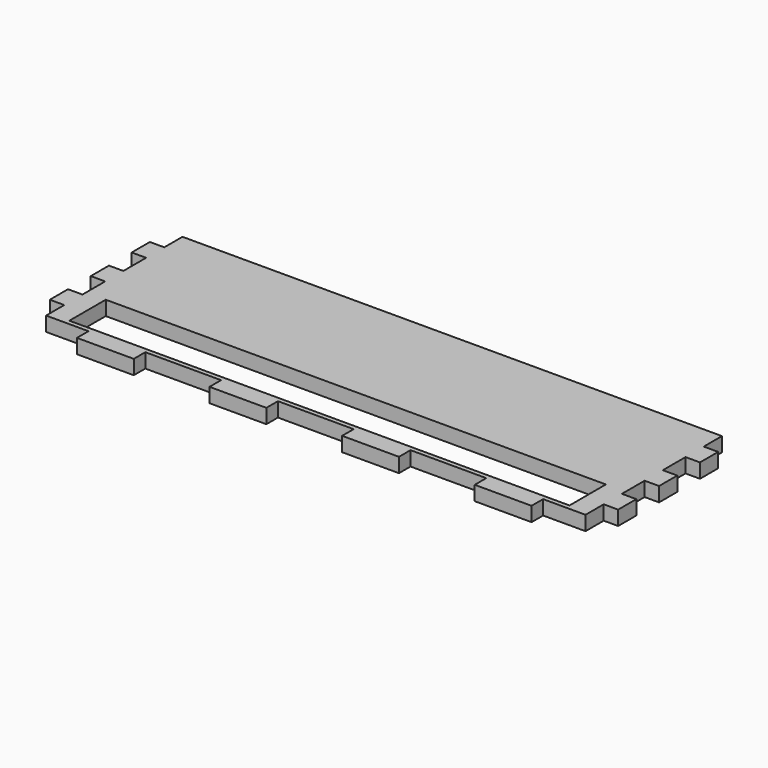
from build123d import *

# Parameters (mm, degrees)
F0_W     = 250
F0_H     = 75
F1_DEPTH = 6.35
F2_W     = 25
F2_H     = 6.35
F3_DEPTH = 6.35
F4_W     = 220
F4_H     = 20
F5_DEPTH = 25
F6_W     = 6.35
F6_H     = 10
F6_H_2   = 12.5
F6_H_3   = 16.35
F7_DEPTH = 6.35


# Not quite as in the source:
# - a length typed as a fraction of an inch, garbled in the dataset ("3 / 203.2 mm" for 3/8 in), is restored


with BuildPart() as f1:
    # F0 (on Top) → F1 (new body)
    with BuildSketch(Plane.XY):
        Rectangle(F0_W, F0_H)
    extrude(amount=F1_DEPTH)

    # F2 (on face) → F3 (join, through all)
    with BuildSketch(Plane.XY.offset(6.35)):
        with Locations((-87.5, -40.675)):
            Rectangle(F2_W, F2_H)
        with Locations((-29.17, -40.675)):
            Rectangle(F2_W, F2_H)
        with Locations((29.16, -40.675)):
            Rectangle(F2_W, F2_H)
        with Locations((87.49, -40.675)):
            Rectangle(F2_W, F2_H)
    extrude(amount=-F3_DEPTH)

    # F4 (on face) → F5 (cut)
    with BuildSketch(Plane.XY.offset(6.35)):
        with Locations((0, -25.5)):
            Rectangle(F4_W, F4_H)
    extrude(amount=-F5_DEPTH, mode=Mode.SUBTRACT)

    # F6 (on face) → F7 (cut, through all)
    with BuildSketch(Plane.XY.offset(6.35)):
        with Locations((121.825, 32.5)):
            Rectangle(F6_W, F6_H)
        with Locations((121.825, 11.25)):
            Rectangle(F6_W, F6_H_2)
        with Locations((121.825, -11.25)):
            Rectangle(F6_W, F6_H_2)
        with Locations((121.825, -35.675)):
            Rectangle(F6_W, F6_H_3)
        with Locations((-121.825, -35.675)):
            Rectangle(F6_W, F6_H_3)
        with Locations((-121.825, 32.5)):
            Rectangle(F6_W, F6_H)
        with Locations((-121.825, 11.25)):
            Rectangle(F6_W, F6_H_2)
        with Locations((-121.825, -11.25)):
            Rectangle(F6_W, F6_H_2)
    extrude(amount=-F7_DEPTH, mode=Mode.SUBTRACT)


solid = f1.part
